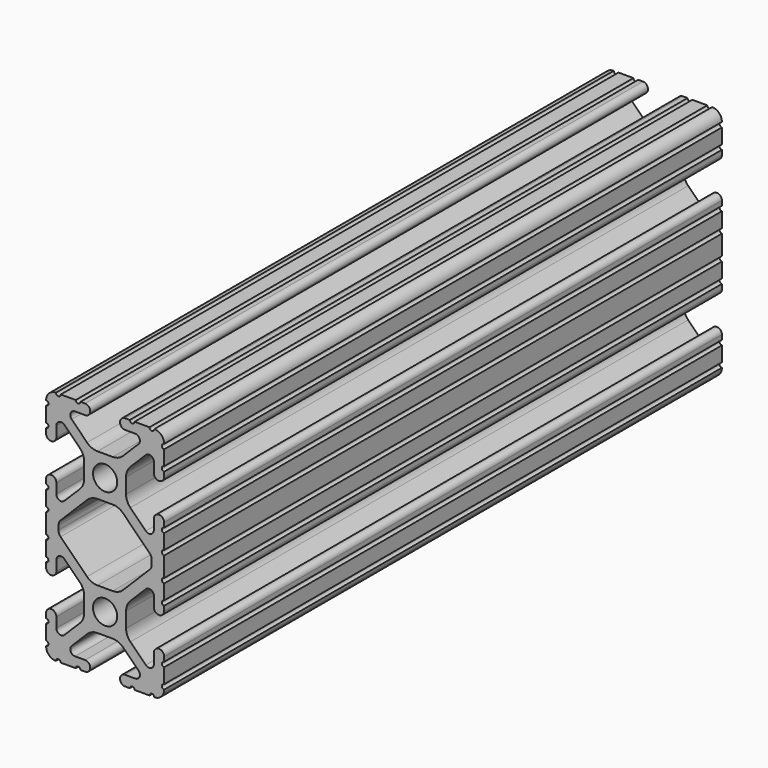
from build123d import *

# Parameters (mm, degrees)
F1_DEPTH = 150


# Not quite as in the source:
# - ends of sketch curves that miss each other by under 0.0002 mm in the source are joined


with BuildPart() as f1:
    # F0 (on Front) → F1 (new body)
    with BuildSketch(Plane.XZ):
        with BuildLine():
            ThreePointArc((-12.6999998568, 23.2791116031), (-12.1919492, 22.76475), (-12.6999998568, 22.2503883969))
            Line((-12.6999998568, 22.2503883969), (-12.7, 19.0246))
            ThreePointArc((-12.7, 19.0246), (-12.192, 18.5166), (-12.7, 18.0086))
            Line((-12.7, 18.0086), (-12.7, 17.0023028))
            ThreePointArc((-12.7, 17.0023028), (-11.5951, 15.8974028), (-10.4902, 17.0023028))
            Line((-10.4902, 17.0023028), (-10.4902, 19.1747902))
            ThreePointArc((-10.4902, 19.1747902), (-9.8630063673, 20.113451805), (-8.7557795103, 19.8932106897))
            Line((-8.7557795103, 19.8932106897), (-5.4384448, 16.5758622))
            ThreePointArc((-5.4384448, 16.5758622), (-4.7501824843, 15.5458268978), (-4.5085, 14.330807))
            Line((-4.5085, 14.330807), (-4.5085, 11.069193))
            ThreePointArc((-4.5085, 11.069193), (-4.7501824843, 9.8541731022), (-5.4384359697, 8.8241289697))
            Line((-5.4384359697, 8.8241289697), (-8.7557864, 5.5067962))
            ThreePointArc((-8.7557864, 5.5067962), (-9.8630063673, 5.286548195), (-10.4902, 6.2252098))
            Line((-10.4902, 6.2252098), (-10.4902, 8.3976972))
            ThreePointArc((-10.4902, 8.3976972), (-11.5951, 9.5025972), (-12.7, 8.3976972))
            Line((-12.7, 8.3976972), (-12.7, 7.3914))
            ThreePointArc((-12.7, 7.3914), (-12.192, 6.8834), (-12.7, 6.3754))
            Line((-12.7, 6.3754), (-12.7, 3.1496))
            ThreePointArc((-12.7, 3.1496), (-12.192, 2.6416), (-12.7, 2.1336))
            Line((-12.7, 2.1336), (-12.7, -2.1336))
            ThreePointArc((-12.7, -2.1336), (-12.192, -2.6416), (-12.7, -3.1496))
            Line((-12.7, -3.1496), (-12.7, -6.3754))
            ThreePointArc((-12.7, -6.3754), (-12.192, -6.8834), (-12.7, -7.3914))
            Line((-12.7, -7.3914), (-12.7, -8.3976972))
            ThreePointArc((-12.7, -8.3976972), (-11.5951, -9.5025972), (-10.4902, -8.3976972))
            Line((-10.4902, -8.3976972), (-10.4902, -6.2252098))
            ThreePointArc((-10.4902, -6.2252098), (-9.8630063673, -5.286548195), (-8.7557795103, -5.5067893103))
            Line((-8.7557795103, -5.5067893103), (-5.4384448, -8.8241378))
            ThreePointArc((-5.4384448, -8.8241378), (-4.7501824843, -9.8541731022), (-4.5085, -11.069193))
            Line((-4.5085, -11.069193), (-4.5085, -14.330807))
            ThreePointArc((-4.5085, -14.330807), (-4.7501824843, -15.5458268978), (-5.4384359697, -16.5758710303))
            Line((-5.4384359697, -16.5758710303), (-8.7557864, -19.8932038))
            ThreePointArc((-8.7557864, -19.8932038), (-9.8630063673, -20.113451805), (-10.4902, -19.1747902))
            Line((-10.4902, -19.1747902), (-10.4902, -17.0023028))
            ThreePointArc((-10.4902, -17.0023028), (-11.5951, -15.8974028), (-12.7, -17.0023028))
            Line((-12.7, -17.0023028), (-12.7, -18.0086))
            ThreePointArc((-12.7, -18.0086), (-12.192, -18.5166), (-12.7, -19.0246))
            Line((-12.7, -19.0246), (-12.7, -22.2504))
            ThreePointArc((-12.7, -22.2504), (-12.1919492, -22.76475), (-12.6999998568, -23.2791116031))
            ThreePointArc((-12.6999998568, -23.2791116031), (-12.0825733161, -24.7825733161), (-10.579099926, -25.4000122396))
            ThreePointArc((-10.579099926, -25.4000122396), (-10.06475, -24.8919492), (-9.5503883969, -25.3999998568))
            Line((-9.5503883969, -25.3999998568), (-6.3246, -25.4))
            ThreePointArc((-6.3246, -25.4), (-5.8166, -24.892), (-5.3086, -25.4))
            Line((-5.3086, -25.4), (-4.3023028, -25.4))
            ThreePointArc((-4.3023028, -25.4), (-3.1974028, -24.2951), (-4.3023028, -23.1902))
            Line((-4.3023028, -23.1902), (-6.4747902, -23.1902))
            ThreePointArc((-6.4747902, -23.1902), (-7.413451805, -22.5630063673), (-7.1932106897, -21.4557795103))
            Line((-7.1932106897, -21.4557795103), (-3.8758622, -18.1384448))
            ThreePointArc((-3.8758622, -18.1384448), (-2.8458268978, -17.4501824843), (-1.630807, -17.2085))
            Line((-1.630807, -17.2085), (1.630807, -17.2085))
            ThreePointArc((1.630807, -17.2085), (2.8458268978, -17.4501824843), (3.8758710303, -18.1384359697))
            Line((3.8758710303, -18.1384359697), (7.1932038, -21.4557864))
            ThreePointArc((7.1932038, -21.4557864), (7.413451805, -22.5630063673), (6.4747902, -23.1902))
            Line((6.4747902, -23.1902), (4.3023028, -23.1902))
            ThreePointArc((4.3023028, -23.1902), (3.1974028, -24.2951), (4.3023028, -25.4))
            Line((4.3023028, -25.4), (5.3086, -25.4))
            ThreePointArc((5.3086, -25.4), (5.8166, -24.892), (6.3246, -25.4))
            Line((6.3246, -25.4), (9.5504, -25.4))
            ThreePointArc((9.5504, -25.4), (10.06475, -24.8919492), (10.5791116031, -25.3999998568))
            ThreePointArc((10.5791116031, -25.3999998568), (12.0825733161, -24.7825733161), (12.7000122396, -23.279099926))
            ThreePointArc((12.7000122396, -23.279099926), (12.1919492, -22.76475), (12.6999998568, -22.2503883969))
            Line((12.6999998568, -22.2503883969), (12.7, -19.0246))
            ThreePointArc((12.7, -19.0246), (12.192, -18.5166), (12.7, -18.0086))
            Line((12.7, -18.0086), (12.7, -17.0023028))
            ThreePointArc((12.7, -17.0023028), (11.5951, -15.8974028), (10.4902, -17.0023028))
            Line((10.4902, -17.0023028), (10.4902, -19.1747902))
            ThreePointArc((10.4902, -19.1747902), (9.8630063673, -20.113451805), (8.7557795103, -19.8932106897))
            Line((8.7557795103, -19.8932106897), (5.4384448, -16.5758622))
            ThreePointArc((5.4384448, -16.5758622), (4.7501824843, -15.5458268978), (4.5085, -14.330807))
            Line((4.5085, -14.330807), (4.5085, -11.069193))
            ThreePointArc((4.5085, -11.069193), (4.7501824843, -9.8541731022), (5.4384359697, -8.8241289697))
            Line((5.4384359697, -8.8241289697), (8.7557864, -5.5067962))
            ThreePointArc((8.7557864, -5.5067962), (9.8630063673, -5.286548195), (10.4902, -6.2252098))
            Line((10.4902, -6.2252098), (10.4902, -8.3976972))
            ThreePointArc((10.4902, -8.3976972), (11.5951, -9.5025972), (12.7, -8.3976972))
            Line((12.7, -8.3976972), (12.7, -7.3914))
            ThreePointArc((12.7, -7.3914), (12.192, -6.8834), (12.7, -6.3754))
            Line((12.7, -6.3754), (12.7, -3.1496))
            ThreePointArc((12.7, -3.1496), (12.192, -2.6416), (12.7, -2.1336))
            Line((12.7, -2.1336), (12.7, 2.1336))
            ThreePointArc((12.7, 2.1336), (12.192, 2.6416), (12.7, 3.1496))
            Line((12.7, 3.1496), (12.7, 6.3754))
            ThreePointArc((12.7, 6.3754), (12.192, 6.8834), (12.7, 7.3914))
            Line((12.7, 7.3914), (12.7, 8.3976972))
            ThreePointArc((12.7, 8.3976972), (11.5951, 9.5025972), (10.4902, 8.3976972))
            Line((10.4902, 8.3976972), (10.4902, 6.2252098))
            ThreePointArc((10.4902, 6.2252098), (9.8630063673, 5.286548195), (8.7557795103, 5.5067893103))
            Line((8.7557795103, 5.5067893103), (5.4384448, 8.8241378))
            ThreePointArc((5.4384448, 8.8241378), (4.7501824843, 9.8541731022), (4.5085, 11.069193))
            Line((4.5085, 11.069193), (4.5085, 14.330807))
            ThreePointArc((4.5085, 14.330807), (4.7501824843, 15.5458268978), (5.4384359697, 16.5758710303))
            Line((5.4384359697, 16.5758710303), (8.7557864, 19.8932038))
            ThreePointArc((8.7557864, 19.8932038), (9.8630063673, 20.113451805), (10.4902, 19.1747902))
            Line((10.4902, 19.1747902), (10.4902, 17.0023028))
            ThreePointArc((10.4902, 17.0023028), (11.5951, 15.8974028), (12.7, 17.0023028))
            Line((12.7, 17.0023028), (12.7, 18.0086))
            ThreePointArc((12.7, 18.0086), (12.192, 18.5166), (12.7, 19.0246))
            Line((12.7, 19.0246), (12.7, 22.2504))
            ThreePointArc((12.7, 22.2504), (12.1919492, 22.76475), (12.6999998568, 23.2791116031))
            ThreePointArc((12.6999998568, 23.2791116031), (12.0825733161, 24.7825733161), (10.579099926, 25.4000122396))
            ThreePointArc((10.579099926, 25.4000122396), (10.06475, 24.8919492), (9.5503883969, 25.3999998568))
            Line((9.5503883969, 25.3999998568), (6.3246, 25.4))
            ThreePointArc((6.3246, 25.4), (5.8166, 24.892), (5.3086, 25.4))
            Line((5.3086, 25.4), (4.3023028, 25.4))
            ThreePointArc((4.3023028, 25.4), (3.1974028, 24.2951), (4.3023028, 23.1902))
            Line((4.3023028, 23.1902), (6.4747902, 23.1902))
            ThreePointArc((6.4747902, 23.1902), (7.413451805, 22.5630063673), (7.1932106897, 21.4557795103))
            Line((7.1932106897, 21.4557795103), (3.8758622, 18.1384448))
            ThreePointArc((3.8758622, 18.1384448), (2.8458268978, 17.4501824843), (1.630807, 17.2085))
            Line((1.630807, 17.2085), (-1.630807, 17.2085))
            ThreePointArc((-1.630807, 17.2085), (-2.8458268978, 17.4501824843), (-3.8758710303, 18.1384359697))
            Line((-3.8758710303, 18.1384359697), (-7.1932038, 21.4557864))
            ThreePointArc((-7.1932038, 21.4557864), (-7.413451805, 22.5630063673), (-6.4747902, 23.1902))
            Line((-6.4747902, 23.1902), (-4.3023028, 23.1902))
            ThreePointArc((-4.3023028, 23.1902), (-3.1974028, 24.2951), (-4.3023028, 25.4))
            Line((-4.3023028, 25.4), (-5.3086, 25.4))
            ThreePointArc((-5.3086, 25.4), (-5.8166, 24.892), (-6.3246, 25.4))
            Line((-6.3246, 25.4), (-9.5504, 25.4))
            ThreePointArc((-9.5504, 25.4), (-10.06475, 24.8919492), (-10.5791116031, 25.3999998568))
            ThreePointArc((-10.5791116031, 25.3999998568), (-12.0825733161, 24.7825733161), (-12.6999998568, 23.2791116031))
        make_face()
        with BuildLine():
            ThreePointArc((-2.6035, -12.7), (0, -10.0965), (2.6035, -12.7))
            ThreePointArc((2.6035, -12.7), (0, -15.3035), (-2.6035, -12.7))
        make_face(mode=Mode.SUBTRACT)
        with BuildLine():
            ThreePointArc((-10.033, 0.45212), (-9.9131254878, 1.0547698693), (-9.571751759, 1.565671759))
            Line((-9.571751759, 1.565671759), (-3.8758622, 7.2615552))
            ThreePointArc((-3.8758622, 7.2615552), (-2.8458268978, 7.9498175157), (-1.630807, 8.1915))
            Line((-1.630807, 8.1915), (1.630807, 8.1915))
            ThreePointArc((1.630807, 8.1915), (2.8458268978, 7.9498175157), (3.8758710303, 7.2615640303))
            Line((3.8758710303, 7.2615640303), (9.5717614, 1.5656814))
            ThreePointArc((9.5717614, 1.5656814), (9.9131254878, 1.0547698693), (10.033, 0.45212))
            Line((10.033, 0.45212), (10.033, -0.45212))
            ThreePointArc((10.033, -0.45212), (9.9131254878, -1.0547698693), (9.571751759, -1.565671759))
            Line((9.571751759, -1.565671759), (3.8758622, -7.2615552))
            ThreePointArc((3.8758622, -7.2615552), (2.8458268978, -7.9498175157), (1.630807, -8.1915))
            Line((1.630807, -8.1915), (-1.630807, -8.1915))
            ThreePointArc((-1.630807, -8.1915), (-2.8458268978, -7.9498175157), (-3.8758710303, -7.2615640303))
            Line((-3.8758710303, -7.2615640303), (-9.5717614, -1.5656814))
            ThreePointArc((-9.5717614, -1.5656814), (-9.9131254878, -1.0547698693), (-10.033, -0.45212))
            Line((-10.033, -0.45212), (-10.033, 0.45212))
        make_face(mode=Mode.SUBTRACT)
        with BuildLine():
            ThreePointArc((-2.6035, 12.7), (0, 15.3035), (2.6035, 12.7))
            ThreePointArc((2.6035, 12.7), (0, 10.0965), (-2.6035, 12.7))
        make_face(mode=Mode.SUBTRACT)
    extrude(amount=F1_DEPTH)


solid = f1.part
